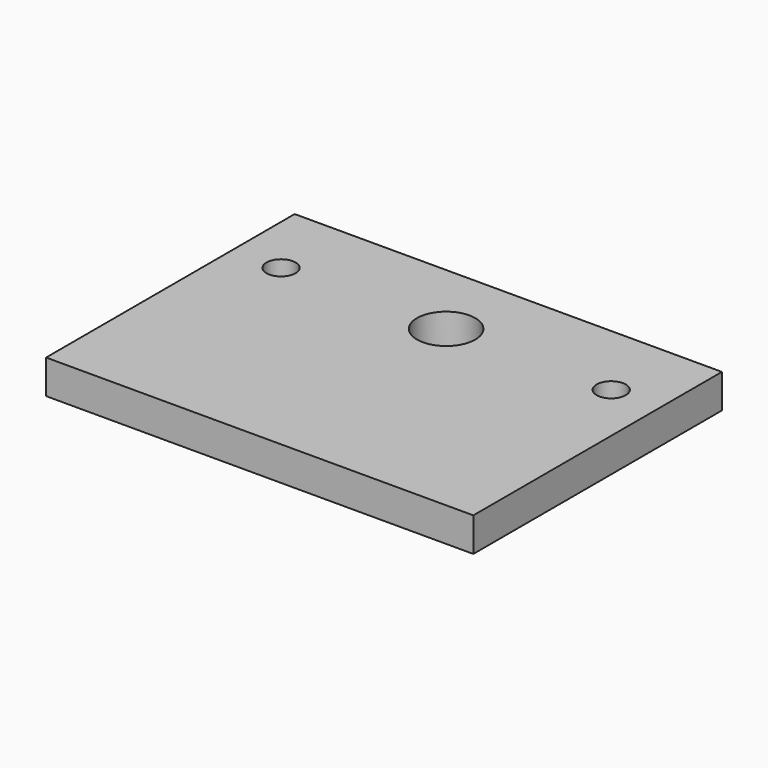
from build123d import *

# Parameters (mm, degrees)
F0_W     = 279.4
F0_H     = 203.2
F1_DEPTH = 22.225
F2_R     = 19.05
F2_R_2   = 9.525
F3_DEPTH = 22.225


# Not quite as in the source:
# - a length typed as a fraction of an inch, garbled in the dataset ("3 / 203.2 mm" for 3/8 in), is restored


with BuildPart() as f1:
    # F0 (on Top) → F1 (new body)
    with BuildSketch(Plane.XY):
        with Locations((139.7, 101.6)):
            Rectangle(F0_W, F0_H)
    extrude(amount=F1_DEPTH)

    # F2 (on face) → F3 (cut)
    with BuildSketch(Plane.XY.offset(22.225)):
        with Locations((139.7, 152.4)):
            Circle(F2_R)
        with Locations((247.65, 152.4)):
            Circle(F2_R_2)
        with Locations((31.75, 152.4)):
            Circle(F2_R_2)
    extrude(amount=-F3_DEPTH, mode=Mode.SUBTRACT)


solid = f1.part
